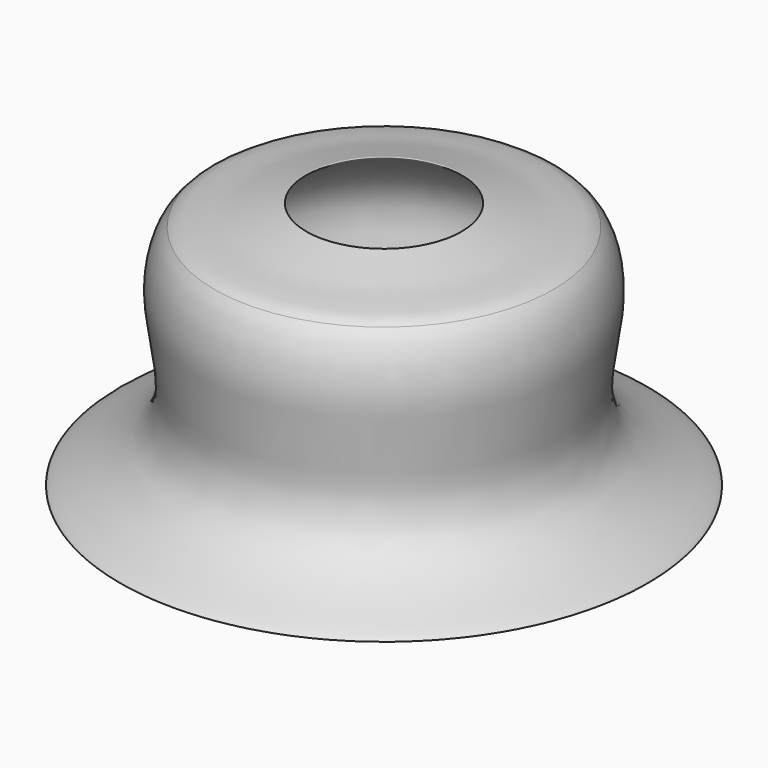
from build123d import *


with BuildPart() as f1:
    # F0 (on Front) → F1 (revolve)
    with BuildSketch(Plane.XZ):
        with BuildLine():
            add(Edge.make_bspline(
                [(0, -46.9601638615), (-0.1644221631, -44.9527123064), (-27.9406439589, -44.6564960234), (-47.9396424125, -37.5760966023), (-51.9808322711, -22.8963117687), (-52.4720088253, -6.7953983045), (-60.8022420464, 21.8437540326), (-11.7780718612, 44.9503437178), (-42.950100772, 34.4784992999), (-51.6021613881, 35.5853695548), (-54.7500066459, 32.9694785178)],
                knots=[0.5022716076, 0.5022716076, 0.5022716076, 0.5022716076, 0.5717592736, 0.6375068936, 0.6866049142, 0.7422789362, 0.8139616294, 0.8926315738, 0.9486421437, 1, 1, 1, 1], degree=3))
            add(Edge.make_bspline(
                [(-54.7500066459, 32.9694785178), (-58.6899024453, 29.6953855226), (-64.2038451711, 10.7572609295), (-48.5936523325, -28.5147149371), (-103.6728210941, -44.065006878), (-49.1703059971, -38.6694163896), (-34.3768944316, -51.9355015537), (-22.9473425561, -51.9381007606), (-13.6203280279, -52.9857038518), (-0.1148978715, -48.4742812388), (0, -47.031598984)],
                knots=[0, 0, 0, 0, 0.0642803523, 0.1484316484, 0.2213899659, 0.2995449064, 0.3638846004, 0.4065137212, 0.4525567435, 0.5014560924, 0.5014560924, 0.5014560924, 0.5014560924], degree=3))
            Line((0, -47.031598984), (0, -46.9601638615))
        make_face()
    revolve(axis=Axis((0, 0, 3.7805512547), (0, 0, -1)))


solid = f1.part
